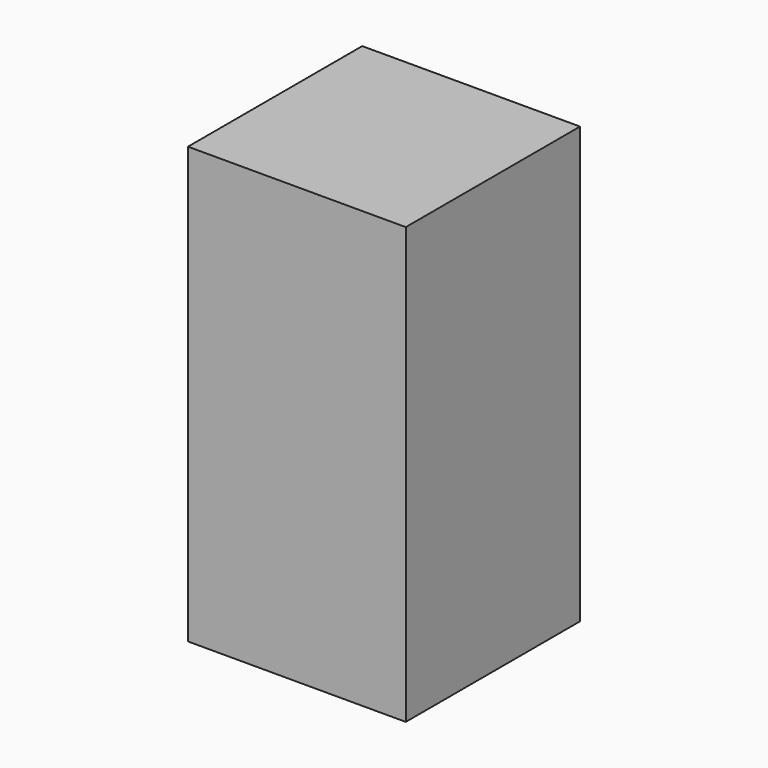
from build123d import *

# Parameters (mm, degrees)
F0_W     = 25
F0_H     = 50
F1_DEPTH = 25
F3_DEPTH = 10


# Not quite as in the source:
# - a feature names something its author has since deleted; it is built from what else it names


with BuildPart() as f1:
    # F0 (on Front) → F1 (new body)
    with BuildSketch(Plane.XZ):
        Rectangle(F0_W, F0_H)
    extrude(amount=F1_DEPTH)

    # F0 (on Front) → F3 (join)
    with BuildSketch(Plane.XZ):
        Rectangle(F0_W, F0_H)
    extrude(amount=F3_DEPTH)


solid = f1.part
